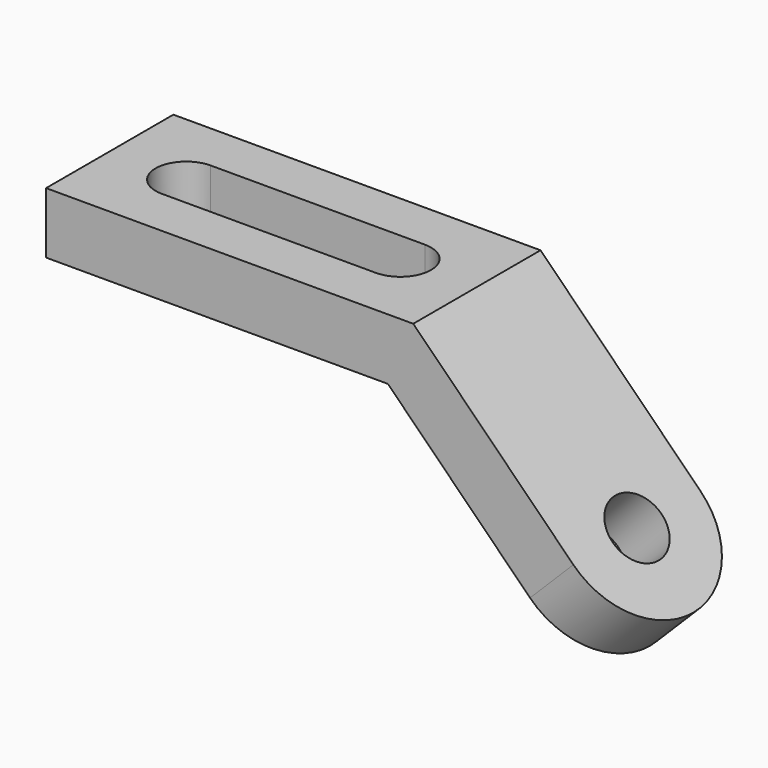
from build123d import *

# Parameters (mm, degrees)
F1_DEPTH = 52
F2_W     = 70
F2_H     = 20
F5_DEPTH = 20
F6_R     = 10
F7_DEPTH = 20
F8_R     = 26
F9_R     = 25.99999


# Not quite as in the source:
# - a fillet or chamfer is up to 0.001 mm smaller than in the source, because OpenCascade refuses the exact size


with BuildPart() as f1:
    # F0 (on Front) → F1 (new body)
    with BuildSketch(Plane.XZ):
        Polygon((91.7157287525, 0), (0, 0), (0, -20), (111.7157287525, -20), align=None)
        Polygon((190.7106781187, -70.7106781187), (120, 0), (120, -20), (111.7157287525, -20), (176.5685424949, -84.8528137424), align=None)
        Polygon((120, 0), (91.7157287525, 0), (111.7157287525, -20), (120, -20), align=None)
    extrude(amount=F1_DEPTH)

    # F2 (on face) + F4 (on face) + F3 (on face) → F5 (cut)
    with BuildSketch(Plane.XY):
        with Locations((60, -26)):
            Rectangle(F2_W, F2_H)
    with BuildSketch(Plane.XY):
        with BuildLine():
            ThreePointArc((95, -36), (102.0710678119, -33.0710678119), (105, -26))
            ThreePointArc((105, -26), (102.0710678119, -18.9289321881), (95, -16))
            Line((95, -16), (95, -36))
        make_face()
    with BuildSketch(Plane.XY):
        with BuildLine():
            Line((25, -36), (25, -16))
            ThreePointArc((25, -16), (15, -26), (25, -36))
        make_face()
    extrude(amount=-F5_DEPTH, mode=Mode.SUBTRACT)

    # F6 (on face) → F7 (cut)
    with BuildSketch(Plane(origin=(60, 0, 60), x_dir=(0.7071067812, 0, -0.7071067812), z_dir=(0.7071067812, 0, 0.7071067812))):
        with Locations((158.8528137424, -26)):
            Circle(F6_R)
    extrude(amount=-F7_DEPTH, mode=Mode.SUBTRACT)

    # F8
    f8_edges = [f1.edges().sort_by_distance(p)[0] for p in [
        (183.63961, -52, -77.781746),
    ]]
    fillet(f8_edges, radius=F8_R)

    # F9 (radius 26 in the source; OpenCascade refuses exactly that, so slightly less here)
    f9_edges = [f1.edges().sort_by_distance(p)[0] for p in [
        (183.63961, 0, -77.781746),
    ]]
    fillet(f9_edges, radius=F9_R)


solid = f1.part
